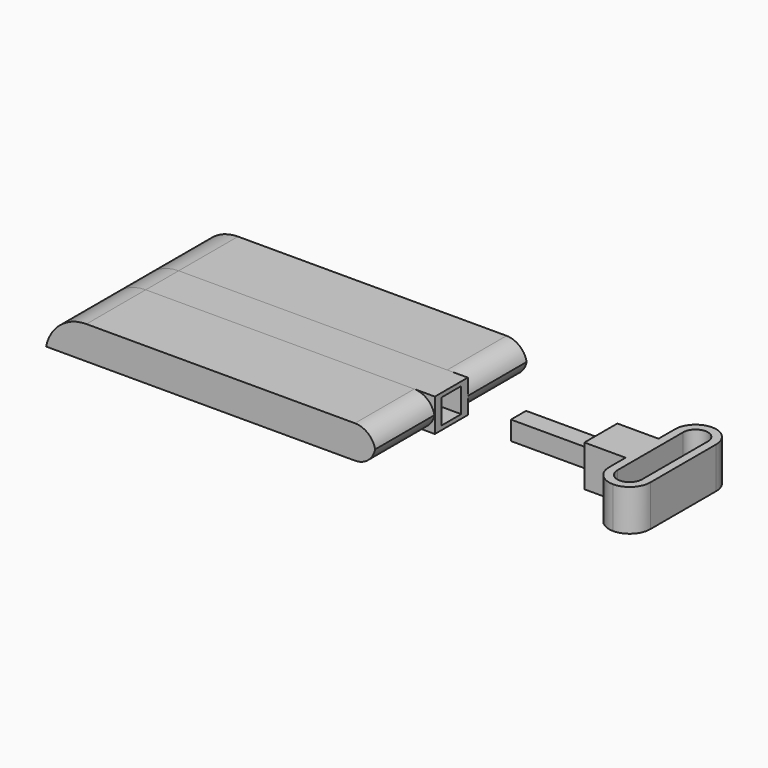
from build123d import *

# Parameters (mm, degrees)
F0_W          = 9
F0_H          = 4
F1_DEPTH      = 40
F0_W_2        = 5
F2_DEPTH      = 40
F3_W          = 3
F3_H          = 3
F4_DEPTH      = 10
F5_T1_DEPTH   = 33.4948974279
F5_2_T1_DEPTH = 33.4948974279
F5_3_T1_DEPTH = 29.4948974279
F6_T1_DEPTH   = 21.5
F6_2_T1_DEPTH = 21.5
F7_W          = 1
F7_H          = 10
F8_DEPTH      = 5
F9_D          = 3
F10_W         = 2.3
F10_H         = 2.3
F11_DEPTH     = 10
F12_R         = 2.49999


# Not quite as in the source:
# - a fillet or chamfer that OpenCascade refuses, or shapes differently, is made with other operations: its cross-section is extruded or revolved along the edge and cut away or added
# - a fillet or chamfer is up to 0.001 mm smaller than in the source, because OpenCascade refuses the exact size


with BuildPart() as f1:
    # F0 (on Right) → F1 (new body)
    with BuildSketch(Plane.YZ):
        with Locations((-4.5, 2)):
            Rectangle(F0_W, F0_H)
    extrude(amount=F1_DEPTH)

    # F5: fillet of radius 5 on 1 edges, made by hand

    # F5_s2 → F5_t1 (cut)
    with BuildSketch(Plane.XZ.offset(-12.2474487139)):
        with BuildLine():
            ThreePointArc((4.8989794856, 4), (1.7367018254, 2.8729833462), (0, 0))
            Line((0, 0), (0, 4))
            Line((0, 4), (4.8989794856, 4))
        make_face()
    extrude(amount=F5_T1_DEPTH, mode=Mode.SUBTRACT)

    # F6: fillet of radius 2.5 on 2 edges, made by hand

    # F6_s2 → F6_t1 (cut)
    with BuildSketch(Plane.XZ.offset(-6.25)):
        with BuildLine():
            ThreePointArc((40, 1.5), (39.267766953, 3.267766953), (37.5, 4))
            Line((37.5, 4), (40, 4))
            Line((40, 4), (40, 1.5))
        make_face()
        with BuildLine():
            ThreePointArc((37.5, 0), (39.267766953, 0.732233047), (40, 2.5))
            Line((40, 2.5), (40, 0))
            Line((40, 0), (37.5, 0))
        make_face()
    extrude(amount=F6_T1_DEPTH, mode=Mode.SUBTRACT)


with BuildPart() as f1b:
    # F0 (on Right) → F1, piece 2 (new body)
    with BuildSketch(Plane.YZ):
        with Locations((9.5, 2)):
            Rectangle(F0_W, F0_H)
    extrude(amount=F1_DEPTH)

    # F5#2: fillet of radius 5 on 1 edges, made by hand

    # F5_2_s2 → F5_2_t1 (cut)
    with BuildSketch(Plane.XZ.offset(-26.2474487139)):
        with BuildLine():
            ThreePointArc((4.8989794856, 4), (1.7367018254, 2.8729833462), (0, 0))
            Line((0, 0), (0, 4))
            Line((0, 4), (4.8989794856, 4))
        make_face()
    extrude(amount=F5_2_T1_DEPTH, mode=Mode.SUBTRACT)

    # F6#2: fillet of radius 2.5 on 2 edges, made by hand

    # F6_2_s2 → F6_2_t1 (cut)
    with BuildSketch(Plane.XZ.offset(-20.25)):
        with BuildLine():
            ThreePointArc((40, 1.5), (39.267766953, 3.267766953), (37.5, 4))
            Line((37.5, 4), (40, 4))
            Line((40, 4), (40, 1.5))
        make_face()
        with BuildLine():
            ThreePointArc((37.5, 0), (39.267766953, 0.732233047), (40, 2.5))
            Line((40, 2.5), (40, 0))
            Line((40, 0), (37.5, 0))
        make_face()
    extrude(amount=F6_2_T1_DEPTH, mode=Mode.SUBTRACT)


with BuildPart() as f2:
    # F0 (on Right) → F2 (new body)
    with BuildSketch(Plane.YZ):
        with Locations((2.5, 2)):
            Rectangle(F0_W_2, F0_H)
    extrude(amount=F2_DEPTH)

    # F3 (on face) → F4 (cut)
    with BuildSketch(Plane.YZ.offset(40)):
        with Locations((2.5, 2)):
            Rectangle(F3_W, F3_H)
    extrude(amount=-F4_DEPTH, mode=Mode.SUBTRACT)

    # F5#3: fillet of radius 5 on 1 edges, made by hand

    # F5_3_s2 → F5_3_t1 (cut)
    with BuildSketch(Plane.XZ.offset(-17.2474487139)):
        with BuildLine():
            ThreePointArc((4.8989794856, 4), (1.7367018254, 2.8729833462), (0, 0))
            Line((0, 0), (0, 4))
            Line((0, 4), (4.8989794856, 4))
        make_face()
    extrude(amount=F5_3_T1_DEPTH, mode=Mode.SUBTRACT)


with BuildPart() as f8:
    # F7 (on Top) → F8 (new body)
    with BuildSketch(Plane.XY):
        Polygon((58.1561289728, 5), (58.1561289728, 0), (63.1561289728, 0), (63.1561289728, -2.5), (64.1561289728, -2.5), (64.1561289728, 7.5), (63.1561289728, 7.5), (63.1561289728, 5), align=None)
        Polygon((64.1561289728, -2.5), (63.1561289728, -2.5), (63.1561289728, -5), (68.1561289728, -5), (68.1561289728, -2.5), (67.1561289728, -2.5), align=None)
        Polygon((63.1561289728, 10), (63.1561289728, 7.5), (64.1561289728, 7.5), (67.1561289728, 7.5), (68.1561289728, 7.5), (68.1561289728, 10), align=None)
        with Locations((67.6561289728, 2.5)):
            Rectangle(F7_W, F7_H)
    extrude(amount=F8_DEPTH)

    # F9 (through all)
    with Locations(Plane(origin=(0, 0, 0), x_dir=(1, 0, 0), z_dir=(0, 0, -1))):
        with Locations((65.6561289728, -7.5), (65.6561289728, 2.5)):
            Hole(F9_D / 2)

    # F10 (on face) → F11 (join)
    with BuildSketch(Plane(origin=(58.1561289728, 0, 0), x_dir=(0, -1, 0), z_dir=(-1, 0, 0))):
        with Locations((-2.5, 2.5)):
            Rectangle(F10_W, F10_H)
    extrude(amount=F11_DEPTH)

    # F12 (radius 2.5 in the source; OpenCascade refuses exactly that, so slightly less here)
    f12_edges = [f8.edges().sort_by_distance(p)[0] for p in [
        (68.156129, 10, 2.5),
        (63.156129, 10, 2.5),
        (68.156129, -5, 2.5),
        (63.156129, -5, 2.5),
    ]]
    fillet(f12_edges, radius=F12_R)


solid = Compound([f1.part, f1b.part, f2.part, f8.part])
